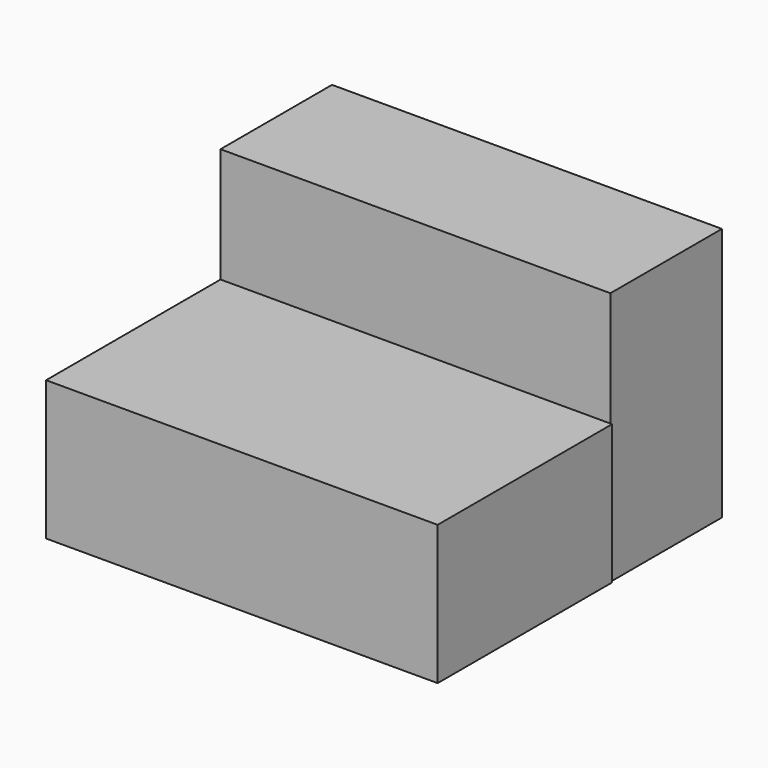
from build123d import *

# Parameters (mm, degrees)
F0_W     = 71.0525270551
F0_H     = 46.3055968285
F1_DEPTH = 25.4
F2_W     = 71.3561698794
F2_H     = 39.7314780116
F3_DEPTH = 25.4


# Not quite as in the source:
# - a feature of the source that left no trace in its solid (it failed there, or was rolled back) is left out


with BuildPart() as f1:
    # F0 (on Front) → F1 (new body)
    with BuildSketch(Plane.XZ):
        with Locations((-6.6801505163, 23.1527984142)):
            Rectangle(F0_W, F0_H)
    extrude(amount=F1_DEPTH)


with BuildPart() as f3:
    # F2 (on face) → F3 (new body)
    with BuildSketch(Plane(origin=(0, 0, 0), x_dir=(1, 0, 0), z_dir=(0, 0, -1))):
        with Locations((-6.5283291042, 45.2657390058)):
            Rectangle(F2_W, F2_H)
    extrude(amount=-F3_DEPTH)


solid = Compound([f1.part, f3.part])
